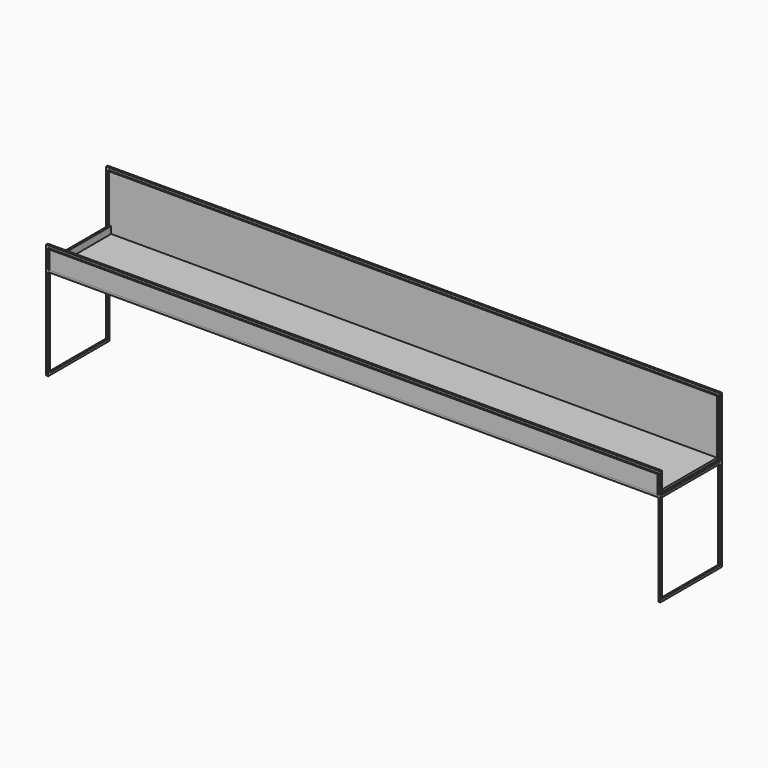
from build123d import *

# Parameters (mm, degrees)
F0_W      = 3657.6
F0_H      = 914.4
F1_DEPTH  = 457.2
F3_DEPTH  = 3657.6
F7_DEPTH  = 1816.1
F8_DEPTH  = 1816.1
F10_DEPTH = 12.7
F11_W     = 12.7
F11_H     = 12.7
F12_DEPTH = 3644.9
F13_W     = 12.7
F13_H     = 12.7
F14_DEPTH = 444.5
F16_DEPTH = 1809.75
F17_DEPTH = 1809.75
F18_W     = 457.2
F18_H     = 53.975
F19_DEPTH = 12.7


with BuildPart() as f1:
    # F0 (on Front) → F1 (new body)
    with BuildSketch(Plane.XZ):
        with Locations((-956.2838003924, 457.2)):
            Rectangle(F0_W, F0_H)
    extrude(amount=F1_DEPTH)

    # F2 (on face) → F3 (cut, through all)
    with BuildSketch(Plane(origin=(-2785.0838003924, 0, 0), x_dir=(0, -1, 0), z_dir=(-1, 0, 0))):
        Polygon((457.2, 558.8), (457.2, 914.4), (12.7, 914.4), (12.7, 12.7), (444.5, 12.7), (444.5, 558.8), align=None)
    extrude(amount=-F3_DEPTH, mode=Mode.SUBTRACT)

    # F6 (on plane+point) → F7 (cut, through all)
    with BuildSketch(Plane.YZ.offset(-956.2838003924)):
        Polygon((178.1790405512, -48.0869802773), (178.1790405512, 901.7), (-187.0097050519, 901.7), (-187.0097050519, 546.1), (-558.2818984985, 546.1), (-558.2818984985, -48.0869802773), align=None)
    extrude(amount=-F7_DEPTH, mode=Mode.SUBTRACT)

    # F6 (on plane+point) → F8 (cut, through all)
    with BuildSketch(Plane.YZ.offset(-956.2838003924)):
        Polygon((178.1790405512, -48.0869802773), (178.1790405512, 901.7), (-187.0097050519, 901.7), (-187.0097050519, 546.1), (-558.2818984985, 546.1), (-558.2818984985, -48.0869802773), align=None)
    extrude(amount=F8_DEPTH, mode=Mode.SUBTRACT)

    # F9 (on face) → F10 (join, through all)
    with BuildSketch(Plane.XZ.offset(457.2)):
        Polygon((-2785.0838003924, 685.8), (-2785.0838003924, 558.8), (-2772.3838003924, 558.8), (-2772.3838003924, 673.1), (859.8161996076, 673.1), (859.8161996076, 558.8), (872.5161996076, 558.8), (872.5161996076, 685.8), align=None)
    extrude(amount=-F10_DEPTH)

    # F11 (on face) → F12 (join, through all)
    with BuildSketch(Plane(origin=(-2785.0838003924, 0, 0), x_dir=(0, -1, 0), z_dir=(-1, 0, 0))):
        with Locations((6.35, 552.45)):
            Rectangle(F11_W, F11_H)
    extrude(amount=-F12_DEPTH)

    # F13 (on face) → F14 (join, through all)
    with BuildSketch(Plane.XZ.offset(457.2)):
        with Locations((-2778.7338003924, 552.45)):
            Rectangle(F13_W, F13_H)
        with Locations((866.1661996076, 552.45)):
            Rectangle(F13_W, F13_H)
        with Locations((-1955.7738003924, 552.45)):
            Rectangle(F13_W, F13_H)
        with Locations((-1132.8138003924, 552.45)):
            Rectangle(F13_W, F13_H)
    extrude(amount=-F14_DEPTH)


with BuildPart() as f16:
    # F15 (on plane+point) → F16 (new body, through all)
    with BuildSketch(Plane.YZ.offset(-956.2838003924)):
        Polygon((0, 558.8), (0, 895.35), (-12.7, 895.35), (-12.7, 571.5), (-444.5, 571.5), (-444.5, 666.75), (-457.2, 666.75), (-457.2, 558.8), align=None)
    extrude(amount=-F16_DEPTH)

    # F15 (on plane+point) → F17 (join, through all)
    with BuildSketch(Plane.YZ.offset(-956.2838003924)):
        Polygon((0, 558.8), (0, 895.35), (-12.7, 895.35), (-12.7, 571.5), (-444.5, 571.5), (-444.5, 666.75), (-457.2, 666.75), (-457.2, 558.8), align=None)
    extrude(amount=F17_DEPTH)

    # F18 (on face) → F19 (join)
    with BuildSketch(Plane(origin=(-2766.0338003924, 0, 0), x_dir=(0, -1, 0), z_dir=(-1, 0, 0))):
        with Locations((228.6, 585.7875)):
            Rectangle(F18_W, F18_H)
    extrude(amount=-F19_DEPTH)


solid = Compound([f1.part, f16.part])
